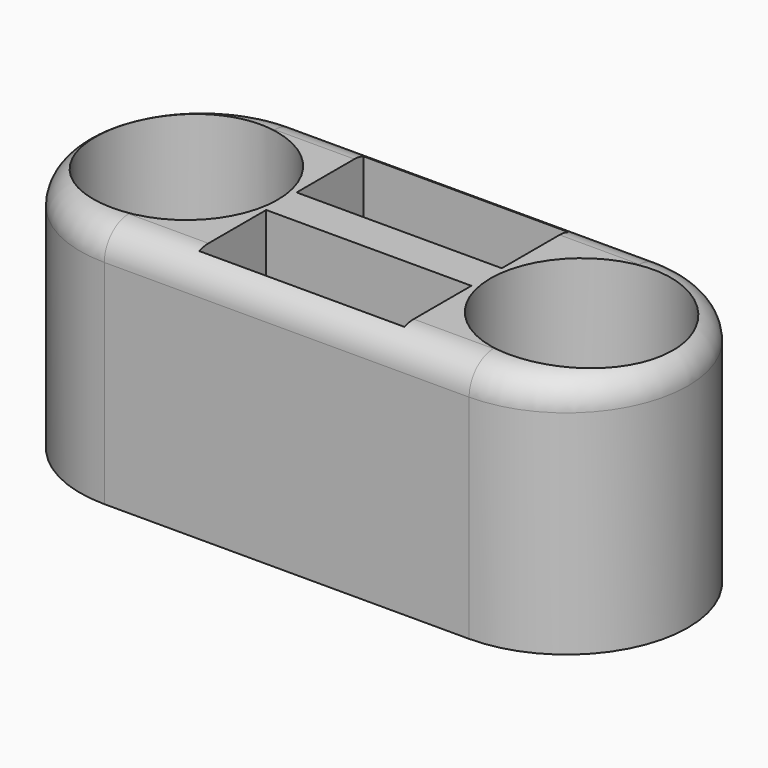
from build123d import *

# Parameters (mm, degrees)
F0_W        = 6.75
F0_H        = 2.75
F0_R        = 1.75
F1_DEPTH    = 8
F2_R        = 3
F2_R_2      = 1.75
F3_DEPTH    = 4
F4_T1_DEPTH = 12
F4_T4_ANGLE = 180
F4_T6_ANGLE = 180


# Not quite as in the source:
# - a fillet or chamfer that OpenCascade refuses, or shapes differently, is made with other operations: its cross-section is extruded or revolved along the edge and cut away or added


with BuildPart() as f1:
    # F0 (on Top) → F1 (new body)
    with BuildSketch(Plane.XY):
        with BuildLine():
            ThreePointArc((6, -4), (10, 0), (6, 4))
            Line((6, 4), (-6, 4))
            ThreePointArc((-6, 4), (-10, 0), (-6, -4))
            Line((-6, -4), (6, -4))
        make_face()
        with Locations((0, -2)):
            Rectangle(F0_W, F0_H, mode=Mode.SUBTRACT)
        with Locations((-6.5, 0)):
            Circle(F0_R, mode=Mode.SUBTRACT)
        with Locations((6.5, 0)):
            Circle(F0_R, mode=Mode.SUBTRACT)
        with Locations((0, 2)):
            Rectangle(F0_W, F0_H, mode=Mode.SUBTRACT)
    extrude(amount=F1_DEPTH)

    # F2 (on face) → F3 (cut)
    with BuildSketch(Plane.XY.offset(8)):
        with Locations((-6.5, 0)):
            Circle(F2_R)
        with Locations((-6.5, 0)):
            Circle(F2_R_2, mode=Mode.SUBTRACT)
        with Locations((6.5, 0)):
            Circle(F2_R)
        with Locations((6.5, 0)):
            Circle(F2_R_2, mode=Mode.SUBTRACT)
    extrude(amount=-F3_DEPTH, mode=Mode.SUBTRACT)

    # F4: fillet of radius 1 on 1 edges, made by hand

    # F4_s2 → F4_t1 (cut)
    with BuildSketch(Plane.YZ.offset(-6)):
        with BuildLine():
            ThreePointArc((-4, 7), (-3.7071067812, 7.7071067812), (-3, 8))
            Line((-3, 8), (-4, 8))
            Line((-4, 8), (-4, 7))
        make_face()
        with BuildLine():
            ThreePointArc((3, 8), (3.7071067812, 7.7071067812), (4, 7))
            Line((4, 7), (4, 8))
            Line((4, 8), (3, 8))
        make_face()
    extrude(amount=F4_T1_DEPTH, mode=Mode.SUBTRACT)

    # F4_s3 → F4_t4 (revolve, cut)
    with BuildSketch(Plane.YZ.offset(6)):
        with BuildLine():
            ThreePointArc((-4, 7), (-3.7071067812, 7.7071067812), (-3, 8))
            Line((-3, 8), (-4, 8))
            Line((-4, 8), (-4, 7))
        make_face()
    revolve(axis=Axis((6, 0, 8), (0, 0, 1)), revolution_arc=F4_T4_ANGLE, mode=Mode.SUBTRACT)

    # F4_s5 → F4_t6 (revolve, cut)
    with BuildSketch(Plane.YZ.offset(-6)):
        with BuildLine():
            ThreePointArc((4, 7), (3.7071067812, 7.7071067812), (3, 8))
            Line((3, 8), (4, 8))
            Line((4, 8), (4, 7))
        make_face()
    revolve(axis=Axis((-6, 0, 8), (0, 0, 1)), revolution_arc=F4_T6_ANGLE, mode=Mode.SUBTRACT)


solid = f1.part
